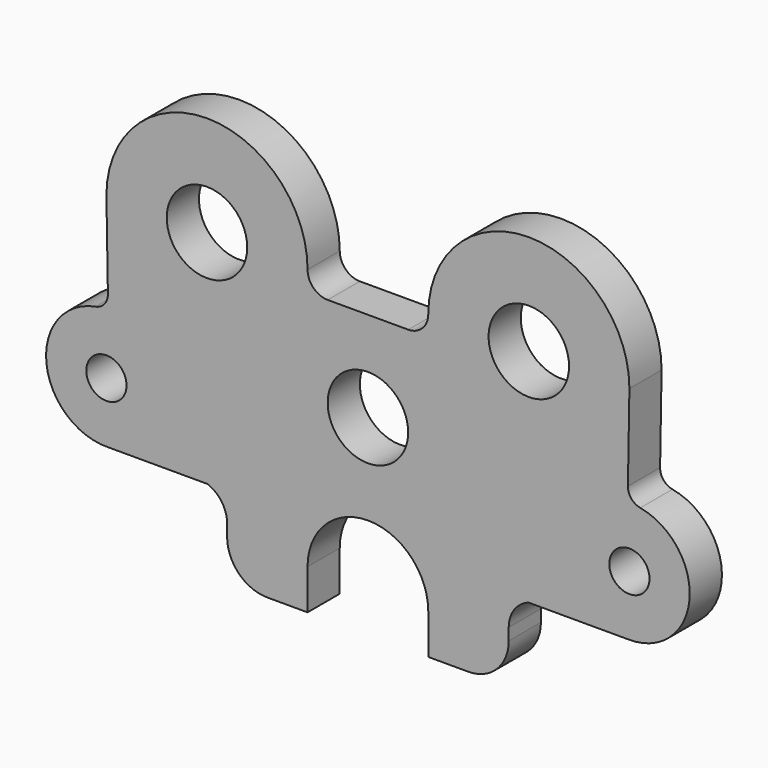
from build123d import *

# Parameters (mm, degrees)
F0_R     = 9.525
F0_R_2   = 12.7
F0_R_3   = 6.35
F1_DEPTH = 6.35
F2_R     = 12.7
F3_R     = 4.7625
F4_R     = 6.34999


# Not quite as in the source:
# - a fillet or chamfer is up to 0.001 mm smaller than in the source, because OpenCascade refuses the exact size


with BuildPart() as f1:
    # F0 (on Front) → F1 (new body, symmetric)
    with BuildSketch(Plane.XZ):
        with BuildLine():
            Line((-19.05, -60.325), (-19.05, -47.625))
            ThreePointArc((-19.05, -47.625), (0, -28.575), (19.05, -47.625))
            Line((19.05, -47.625), (19.05, -60.325))
            Line((19.05, -60.325), (44.45, -60.325))
            Line((44.45, -60.325), (44.45, -43.8458790377))
            ThreePointArc((44.45, -43.8458790377), (46.1544838519, -38.4084943559), (50.6579059691, -34.9171326425))
            Line((50.6579059691, -34.9171326425), (82.0025655956, -34.9171326425))
            ThreePointArc((82.0025655956, -34.9171326425), (101.6, -15.875), (82.0025655956, 3.1671326425))
            Line((82.0025655956, 3.1671326425), (82.55, 34.925))
            ThreePointArc((82.55, 34.925), (50.8, 66.675), (19.05, 34.925))
            Line((19.05, 34.925), (19.05, 28.575))
            Line((19.05, 28.575), (-19.05, 28.575))
            Line((-19.05, 28.575), (-19.05, 34.925))
            ThreePointArc((-19.05, 34.925), (-50.8, 66.675), (-82.55, 34.925))
            Line((-82.55, 34.925), (-82.0025655956, 3.1671326425))
            ThreePointArc((-82.0025655956, 3.1671326425), (-101.6, -15.875), (-82.0025655956, -34.9171326425))
            Line((-82.0025655956, -34.9171326425), (-50.6579059691, -34.9171326425))
            ThreePointArc((-50.6579059691, -34.9171326425), (-46.1544838519, -38.4084943559), (-44.45, -43.8458790377))
            Line((-44.45, -43.8458790377), (-44.45, -60.325))
            Line((-44.45, -60.325), (-19.05, -60.325))
        make_face()
        with Locations((-82.55, -15.875)):
            Circle(F0_R, mode=Mode.SUBTRACT)
        Circle(F0_R_2, mode=Mode.SUBTRACT)
        with Locations((82.55, -15.875)):
            Circle(F0_R, mode=Mode.SUBTRACT)
        with Locations((-50.8, 34.925)):
            Circle(F0_R_2, mode=Mode.SUBTRACT)
        with Locations((50.8, 34.925)):
            Circle(F0_R_2, mode=Mode.SUBTRACT)
        with Locations((82.55, -15.875)):
            Circle(F0_R)
        with Locations((82.55, -15.875)):
            Circle(F0_R_3, mode=Mode.SUBTRACT)
        with Locations((-82.55, -15.875)):
            Circle(F0_R)
        with Locations((-82.55, -15.875)):
            Circle(F0_R_3, mode=Mode.SUBTRACT)
    extrude(amount=F1_DEPTH, both=True)

    # F2
    f2_edges = [f1.edges().sort_by_distance(p)[0] for p in [
        (-44.45, 0, -60.325),
        (44.45, 0, -60.325),
    ]]
    fillet(f2_edges, radius=F2_R)

    # F3
    f3_edges = [f1.edges().sort_by_distance(p)[0] for p in [
        (-82.002566, 0, 3.167133),
        (82.002566, 0, 3.167133),
    ]]
    fillet(f3_edges, radius=F3_R)

    # F4 (radius 6.35 in the source; OpenCascade refuses exactly that, so slightly less here)
    f4_edges = [f1.edges().sort_by_distance(p)[0] for p in [
        (-19.05, 0, 28.575),
        (19.05, 0, 28.575),
    ]]
    fillet(f4_edges, radius=F4_R)


solid = f1.part
